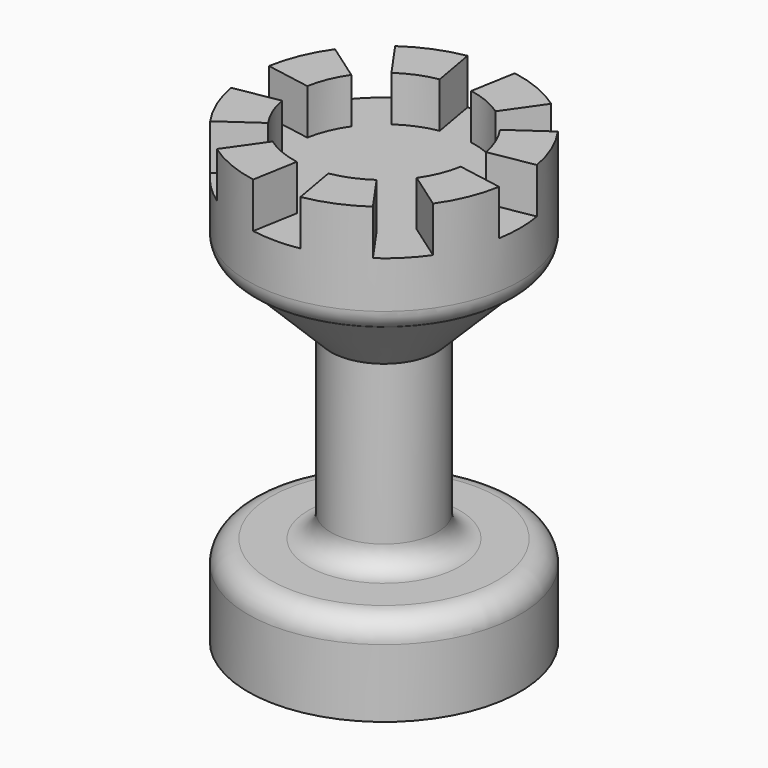
from build123d import *

# Parameters (mm, degrees)
F3_DEPTH = 10
F4_R     = 5
F5_SIZE  = 15


# Not quite as in the source:
# - a fillet or chamfer that OpenCascade refuses, or shapes differently, is made with other operations: its cross-section is extruded or revolved along the edge and cut away or added


with BuildPart() as f1:
    # F0 (on Front) → F1 (revolve)
    with BuildSketch(Plane.XZ):
        Polygon((-30, 0), (0, 0), (0, 90), (-20, 90), (-20, 100), (-30, 100), (-30, 75), (-11.7123959959, 75), (-11.7123959959, 20), (-30, 20), align=None)
    revolve(axis=Axis((0, 0, 45), (0, 0, -1)))

    # F2 (on face) → F3 (cut)
    with BuildSketch(Plane.XY.offset(100)):
        with BuildLine():
            ThreePointArc((-3.2492678477, 18.4275136719), (0, 18.7117877734), (3.2492678477, 18.4275136719))
            Line((3.2492678477, 18.4275136719), (5.5579839553, 31.5208933594))
            ThreePointArc((5.5579839553, 31.5208933594), (0, 32.0071539476), (-5.5579839553, 31.5208933594))
            Line((-5.5579839553, 31.5208933594), (-3.2492678477, 18.4275136719))
        make_face()
        with BuildLine():
            ThreePointArc((-15.3277992068, 10.7326405488), (-13.2312320227, 13.2312320227), (-10.7326405488, 15.3277992068))
            Line((-10.7326405488, 15.3277992068), (-18.358549299, 26.218725588))
            ThreePointArc((-18.358549299, 26.218725588), (-22.6324756028, 22.6324756028), (-26.218725588, 18.358549299))
            Line((-26.218725588, 18.358549299), (-15.3277992068, 10.7326405488))
        make_face()
        with BuildLine():
            ThreePointArc((-18.4275136719, -3.2492678477), (-18.7117877734, 0), (-18.4275136719, 3.2492678477))
            Line((-18.4275136719, 3.2492678477), (-31.5208933594, 5.5579839553))
            ThreePointArc((-31.5208933594, 5.5579839553), (-32.0071539476, 0), (-31.5208933594, -5.5579839553))
            Line((-31.5208933594, -5.5579839553), (-18.4275136719, -3.2492678477))
        make_face()
        with BuildLine():
            ThreePointArc((-10.7326405488, -15.3277992068), (-13.2312320227, -13.2312320227), (-15.3277992068, -10.7326405488))
            Line((-15.3277992068, -10.7326405488), (-26.218725588, -18.358549299))
            ThreePointArc((-26.218725588, -18.358549299), (-22.6324756028, -22.6324756028), (-18.358549299, -26.218725588))
            Line((-18.358549299, -26.218725588), (-10.7326405488, -15.3277992068))
        make_face()
        with BuildLine():
            ThreePointArc((3.2492678477, -18.4275136719), (0, -18.7117877734), (-3.2492678477, -18.4275136719))
            Line((-3.2492678477, -18.4275136719), (-5.5579839553, -31.5208933594))
            ThreePointArc((-5.5579839553, -31.5208933594), (0, -32.0071539476), (5.5579839553, -31.5208933594))
            Line((5.5579839553, -31.5208933594), (3.2492678477, -18.4275136719))
        make_face()
        with BuildLine():
            ThreePointArc((15.3277992068, -10.7326405488), (13.2312320227, -13.2312320227), (10.7326405488, -15.3277992068))
            Line((10.7326405488, -15.3277992068), (18.358549299, -26.218725588))
            ThreePointArc((18.358549299, -26.218725588), (22.6324756028, -22.6324756028), (26.218725588, -18.358549299))
            Line((26.218725588, -18.358549299), (15.3277992068, -10.7326405488))
        make_face()
        with BuildLine():
            ThreePointArc((18.4275136719, 3.2492678477), (18.7117877734, 0), (18.4275136719, -3.2492678477))
            Line((18.4275136719, -3.2492678477), (31.5208933594, -5.5579839553))
            ThreePointArc((31.5208933594, -5.5579839553), (32.0071539476, 0), (31.5208933594, 5.5579839553))
            Line((31.5208933594, 5.5579839553), (18.4275136719, 3.2492678477))
        make_face()
        with BuildLine():
            ThreePointArc((10.7326405488, 15.3277992068), (13.2312320227, 13.2312320227), (15.3277992068, 10.7326405488))
            Line((15.3277992068, 10.7326405488), (26.218725588, 18.358549299))
            ThreePointArc((26.218725588, 18.358549299), (22.6324756028, 22.6324756028), (18.358549299, 26.218725588))
            Line((18.358549299, 26.218725588), (10.7326405488, 15.3277992068))
        make_face()
    extrude(amount=-F3_DEPTH, mode=Mode.SUBTRACT)

    # F4
    f4_edges = [f1.edges().sort_by_distance(p)[0] for p in [
        (11.712396, 0, 20),
        (30, 0, 20),
    ]]
    fillet(f4_edges, radius=F4_R)

    # F5
    f5_edges = [f1.edges().sort_by_distance(p)[0] for p in [
        (11.712396, 0, 75),
    ]]
    chamfer(f5_edges, length=F5_SIZE)

    # F6: fillet of radius 5 on 1 edges, made by hand

    # F6_s1 → F6_t2 (revolve, cut)
    with BuildSketch(Plane.XZ):
        with BuildLine():
            ThreePointArc((-26.7123959959, 75), (-29.0964606662, 76.8307454727), (-30, 79.6976270556))
            Line((-30, 79.6976270556), (-30.1, 79.6976270556))
            Line((-30.1, 79.6976270556), (-30.1, 75))
            Line((-30.1, 75), (-30, 74.9))
            ThreePointArc((-30, 74.9), (-28.3561979979, 74.9), (-26.7466439158, 74.9060474589))
            Line((-26.7466439158, 74.9060474589), (-26.7123959959, 75))
        make_face()
    revolve(axis=Axis((0, 0, 75), (0, 0, -1)), mode=Mode.SUBTRACT)


solid = f1.part
